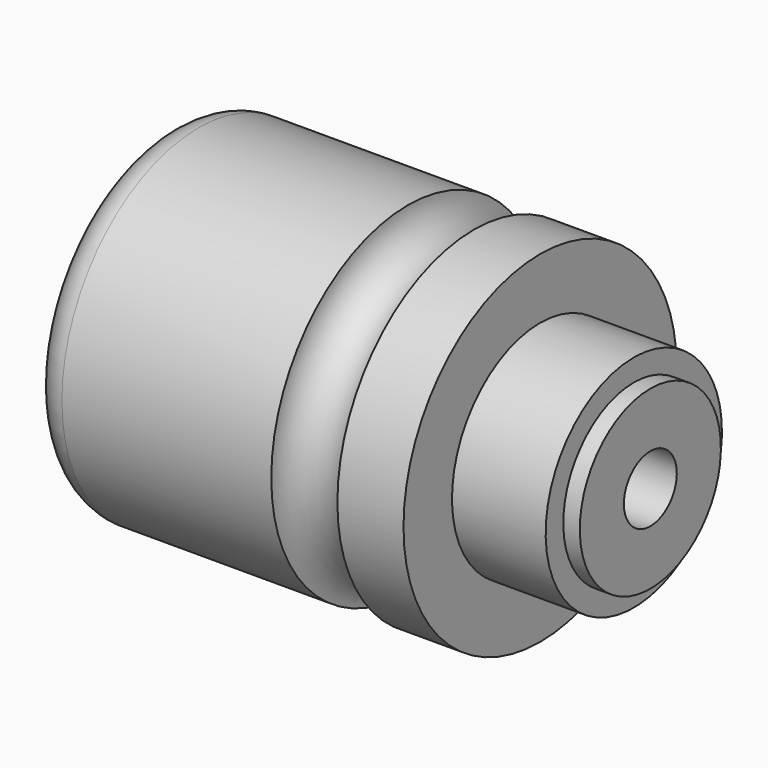
from build123d import *

# Parameters (mm, degrees)
F4_R = 5.99999


# Not quite as in the source:
# - a fillet or chamfer is up to 0.001 mm smaller than in the source, because OpenCascade refuses the exact size


with BuildPart() as f1:
    # F0 (on Front) → F1 (revolve)
    with BuildSketch(Plane.XZ):
        with BuildLine():
            Line((0, 31), (0, 0))
            Line((0, 0), (88, 0))
            Line((88, 0), (88, 16))
            Line((88, 16), (85, 16))
            Line((85, 16), (85, 20))
            Line((85, 20), (68, 20))
            Line((68, 20), (68, 31))
            Line((68, 31), (56, 31))
            ThreePointArc((56, 31), (50, 25), (44, 31))
            Line((44, 31), (0, 31))
        make_face()
    revolve(axis=Axis((68.2048197045, 0, 0), (1, 0, 0)))

    # F2 (on Front) → F3 (revolve, cut)
    with BuildSketch(Plane.XZ):
        Polygon((1.5, 25), (0, 25), (0, 0), (88, 0), (88, 6), (30, 6), (30, 16), (22, 16), (22, 20.5), (19, 20.5), (19, 12.5), (12, 12.5), (12, 16), (1.5, 16), align=None)
    revolve(axis=Axis((-8.4996176884, 0, 0), (-1, 0, 0)), mode=Mode.SUBTRACT)

    # F4 (radius 6 in the source; OpenCascade refuses exactly that, so slightly less here)
    f4_edges = [f1.edges().sort_by_distance(p)[0] for p in [
        (0, 0, -31),
    ]]
    fillet(f4_edges, radius=F4_R)


solid = f1.part
